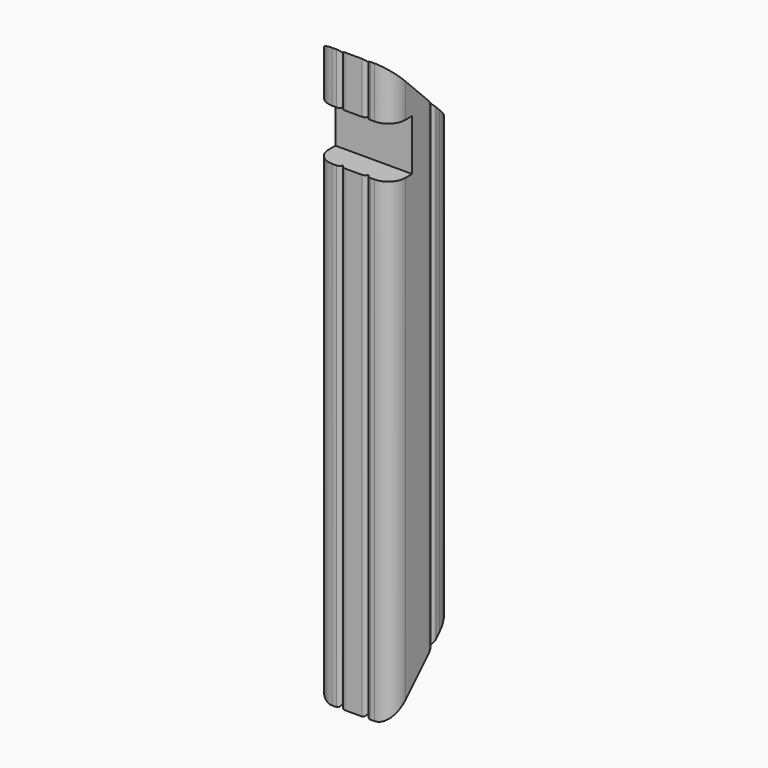
from build123d import *

# Parameters (mm, degrees)
F1_DEPTH = 431.8
F3_DEPTH = 57.151
F4_W     = 12.7
F4_H     = 38.1
F4_W_2   = 6.35
F5_DEPTH = 57.151


# Not quite as in the source:
# - ends of sketch curves that miss each other by under 0.0002 mm in the source are joined


with BuildPart() as f1:
    # F0 (on Top) → F1 (new body)
    with BuildSketch(Plane.XY):
        with BuildLine():
            ThreePointArc((0, 12.7), (3.7197438789, 3.7197438789), (12.7, 0))
            Line((12.7, 0), (15.9004, 0))
            ThreePointArc((15.9004, 0), (18.127503518, 0.922496482), (19.05, 3.1496))
            Line((19.05, 3.1496), (19.05, 34.9504))
            ThreePointArc((19.05, 34.9504), (18.127503518, 37.177503518), (15.9004, 38.1))
            Line((15.9004, 38.1), (3.1496, 38.1))
            ThreePointArc((3.1496, 38.1), (0.922496482, 37.177503518), (0, 34.9504))
            Line((0, 34.9504), (0, 12.7))
        make_face()
        with BuildLine():
            Line((19.05, 34.9504), (19.05, 3.1496))
            ThreePointArc((19.05, 3.1496), (19.972496482, 0.922496482), (22.1996, 0))
            Line((22.1996, 0), (34.9504, 0))
            ThreePointArc((34.9504, 0), (37.177503518, 0.922496482), (38.1, 3.1496))
            Line((38.1, 3.1496), (38.1, 34.9504))
            ThreePointArc((38.1, 34.9504), (37.177503518, 37.177503518), (34.9504, 38.1))
            Line((34.9504, 38.1), (22.1996, 38.1))
            ThreePointArc((22.1996, 38.1), (19.972496482, 37.177503518), (19.05, 34.9504))
        make_face()
        with BuildLine():
            Line((38.1, 34.9504), (38.1, 3.1496))
            ThreePointArc((38.1, 3.1496), (39.022496482, 0.922496482), (41.2496, 0))
            Line((41.2496, 0), (44.45, 0))
            ThreePointArc((44.45, 0), (53.4302561211, 3.7197438789), (57.15, 12.7))
            Line((57.15, 12.7), (57.15, 34.9504))
            ThreePointArc((57.15, 34.9504), (56.227503518, 37.177503518), (54.0004, 38.1))
            Line((54.0004, 38.1), (41.2496, 38.1))
            ThreePointArc((41.2496, 38.1), (39.022496482, 37.177503518), (38.1, 34.9504))
        make_face()
        with BuildLine():
            ThreePointArc((19.0499988437, 41.2496), (19.9724953256, 39.022496482), (22.1995988437, 38.1))
            Line((22.1995988437, 38.1), (34.9504, 38.1))
            Line((34.9504, 38.1), (41.2496, 38.1))
            Line((41.2496, 38.1), (54.0004, 38.1))
            ThreePointArc((54.0004, 38.1), (56.2275023617, 39.022496482), (57.1499988437, 41.2496))
            Line((57.1499988437, 41.2496), (57.1499988437, 44.45))
            ThreePointArc((57.1499988437, 44.45), (53.4302549647, 53.4302561211), (44.4499988437, 57.15))
            Line((44.4499988437, 57.15), (22.1995988437, 57.15))
            ThreePointArc((22.1995988437, 57.15), (19.9724953256, 56.227503518), (19.0499988437, 54.0004))
            Line((19.0499988437, 54.0004), (19.0499988437, 41.2496))
        make_face()
    extrude(amount=F1_DEPTH)

    # F2 (on face) → F3 (cut, through all)
    with BuildSketch(Plane.YZ.offset(57.15)):
        Polygon((57.15, 0), (57.15, 57.15), (0, 0), (12.7, 0), align=None)
        Polygon((12.7, 431.8), (0, 431.8), (57.15, 374.65), (57.15, 431.8), align=None)
    extrude(amount=-F3_DEPTH, mode=Mode.SUBTRACT)

    # F4 (on face) → F5 (cut, through all)
    with BuildSketch(Plane.YZ.offset(57.15)):
        with Locations((6.35, 374.65)):
            Rectangle(F4_W, F4_H)
        with Locations((15.875, 374.65)):
            Rectangle(F4_W_2, F4_H)
    extrude(amount=-F5_DEPTH, mode=Mode.SUBTRACT)


solid = f1.part
